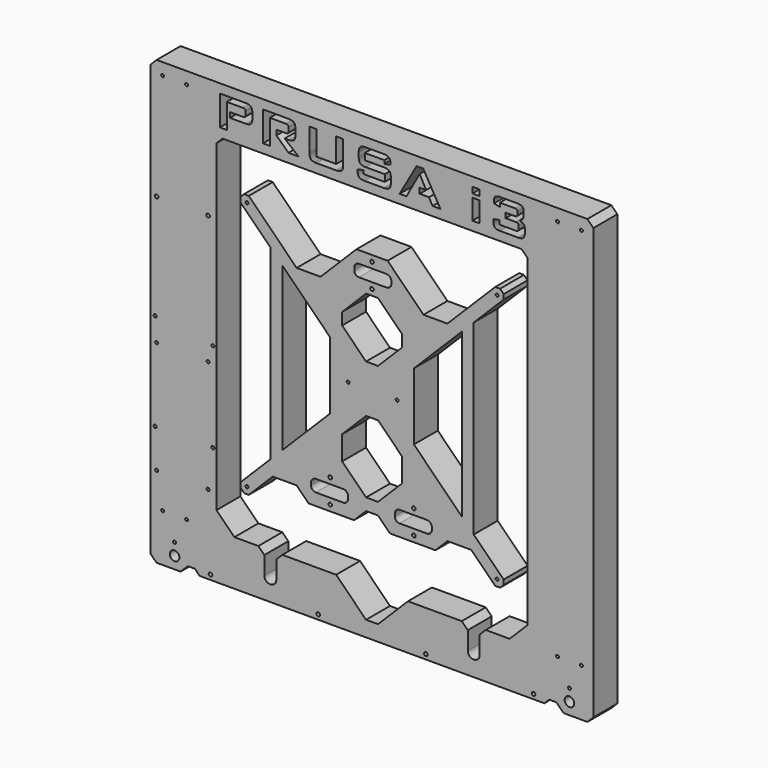
from build123d import *

# Parameters (mm, degrees)
F0_R     = 4
F0_R_2   = 1.2295
F0_R_3   = 1.5
F0_W     = 5.816832
F0_H     = 17
F0_H_2   = 5
F1_DEPTH = 25


# Not quite as in the source:
# - ends of sketch curves that miss each other by under 0.0002 mm in the source are joined


with BuildPart() as f1:
    # F0 (on Front) → F1 (new body)
    with BuildSketch(Plane.XZ):
        Polygon((338.0000003539, 10.00000019), (344.0000003539, 10.00000019), (350.0000003539, 4.00000019), (370.0000003539, 4.00000019), (375.0000003539, 9.00000019), (375.0000003539, 369.00000019), (370.0000003539, 374.00000019), (10.0000003539, 374.00000019), (5.0000003539, 369.00000019), (5.0000003539, 8.80825219), (10.0000003539, 4.00000019), (30.0000003539, 4.00000019), (36.0000003539, 10.00000019), (42.0000003539, 10.00000019), (46.0000003539, 6.00000019), (334.0000003539, 6.00000019), align=None)
        with Locations((25.0000003539, 14.00000019)):
            Circle(F0_R, mode=Mode.SUBTRACT)
        with Locations((25.0000003539, 24.00000019)):
            Circle(F0_R_2, mode=Mode.SUBTRACT)
        with Locations((15.0000003539, 44.00000019)):
            Circle(F0_R_2, mode=Mode.SUBTRACT)
        with Locations((35.0000003539, 44.00000019)):
            Circle(F0_R_2, mode=Mode.SUBTRACT)
        with Locations((55.0000003539, 10.00000019)):
            Circle(F0_R_3, mode=Mode.SUBTRACT)
        with Locations((10.0000003539, 72.00000019)):
            Circle(F0_R_2, mode=Mode.SUBTRACT)
        with Locations((53.0000003539, 72.00000019)):
            Circle(F0_R_2, mode=Mode.SUBTRACT)
        with Locations((145.0000003539, 10.00000019)):
            Circle(F0_R_3, mode=Mode.SUBTRACT)
        with Locations((8.7400003539, 104.00000019)):
            Circle(F0_R_2, mode=Mode.SUBTRACT)
        with Locations((57.0000003539, 104.00000019)):
            Circle(F0_R_2, mode=Mode.SUBTRACT)
        with Locations((10.0000003539, 166.00000019)):
            Circle(F0_R_2, mode=Mode.SUBTRACT)
        with Locations((8.7400003539, 185.28000019)):
            Circle(F0_R_2, mode=Mode.SUBTRACT)
        with Locations((53.0000003539, 166.00000019)):
            Circle(F0_R_2, mode=Mode.SUBTRACT)
        with Locations((57.0000003539, 178.93000019)):
            Circle(F0_R_2, mode=Mode.SUBTRACT)
        with BuildLine():
            Line((60.0000003539, 59.00000019), (60.0000003539, 329.00000019))
            Line((60.0000003539, 329.00000019), (65.0000003539, 334.00000019))
            Line((65.0000003539, 334.00000019), (315.0000003539, 334.00000019))
            Line((315.0000003539, 334.00000019), (320.0000003539, 329.00000019))
            Line((320.0000003539, 329.00000019), (320.0000003539, 59.00000019))
            Line((320.0000003539, 59.00000019), (305.0000003539, 44.00000019))
            Line((305.0000003539, 44.00000019), (285.0000003539, 44.00000019))
            Line((285.0000003539, 44.00000019), (280.0000003539, 39.00000019))
            Line((280.0000003539, 39.00000019), (280.0000003539, 24.00000019))
            ThreePointArc((280.0000003539, 24.00000019), (275.0000003539, 19.00000019), (270.0000003539, 24.00000019))
            Line((270.0000003539, 24.00000019), (270.0000003539, 39.00000019))
            Line((270.0000003539, 39.00000019), (265.0000003539, 44.00000019))
            Line((265.0000003539, 44.00000019), (220.0000003539, 44.00000019))
            Line((220.0000003539, 44.00000019), (195.0000003539, 19.00000019))
            Line((195.0000003539, 19.00000019), (185.0000003539, 19.00000019))
            Line((185.0000003539, 19.00000019), (160.0000003539, 44.00000019))
            Line((160.0000003539, 44.00000019), (115.0000003539, 44.00000019))
            Line((115.0000003539, 44.00000019), (110.0000003539, 39.00000019))
            Line((110.0000003539, 39.00000019), (110.0000003539, 24.00000019))
            ThreePointArc((110.0000003539, 24.00000019), (105.0000003539, 19.00000019), (100.0000003539, 24.00000019))
            Line((100.0000003539, 24.00000019), (100.0000003539, 39.00000019))
            Line((100.0000003539, 39.00000019), (95.0000003539, 44.00000019))
            Line((95.0000003539, 44.00000019), (75.0000003539, 44.00000019))
            Line((75.0000003539, 44.00000019), (65.0000003539, 54.00000019))
            Line((65.0000003539, 54.00000019), (60.0000003539, 59.00000019))
        make_face(mode=Mode.SUBTRACT)
        with Locations((235.0000003539, 10.00000019)):
            Circle(F0_R_3, mode=Mode.SUBTRACT)
        with Locations((325.0000003539, 10.00000019)):
            Circle(F0_R_3, mode=Mode.SUBTRACT)
        with Locations((355.0000003539, 14.00000019)):
            Circle(F0_R, mode=Mode.SUBTRACT)
        with Locations((355.0000003539, 24.00000019)):
            Circle(F0_R_2, mode=Mode.SUBTRACT)
        with Locations((345.0000003539, 44.00000019)):
            Circle(F0_R_2, mode=Mode.SUBTRACT)
        with Locations((365.0000003539, 44.00000019)):
            Circle(F0_R_2, mode=Mode.SUBTRACT)
        with Locations((10.0000003539, 273.50000019)):
            Circle(F0_R_3, mode=Mode.SUBTRACT)
        with Locations((53.0000003539, 273.50000019)):
            Circle(F0_R_3, mode=Mode.SUBTRACT)
        with Locations((15.0000003539, 364.00000019)):
            Circle(F0_R_2, mode=Mode.SUBTRACT)
        with Locations((35.0000003539, 364.00000019)):
            Circle(F0_R_2, mode=Mode.SUBTRACT)
        Polygon((81.6980203539, 362.16831719), (68.6039603539, 362.16831719), (68.6039603539, 341.50000019), (62.8861393539, 341.50000019), (62.8861393539, 366.50000019), (84.2722773539, 366.50000019), (84.7559833539, 366.49198919), (85.2169993539, 366.46803319), (85.6553223539, 366.42805519), (86.0709573539, 366.37209319), (86.4639043539, 366.30018619), (86.8341593539, 366.21225719), (87.1817263539, 366.10834519), (87.5065993539, 365.98844919), (87.8087853539, 365.85257019), (88.0882843539, 365.70070619), (88.3450893539, 365.53286019), (88.5792063539, 365.34899119), (88.7926963539, 365.14746119), (88.9876223539, 364.92651419), (89.1639853539, 364.68611119), (89.3217803539, 364.42629219), (89.4610173539, 364.14705719), (89.5816853539, 363.84840419), (89.6837853539, 363.53029619), (89.7673273539, 363.19281019), (89.8323013539, 362.83586919), (89.8787123539, 362.45951119), (89.9065593539, 362.06373619), (89.9158433539, 361.64850619), (89.9158423539, 356.07920819), (89.9065593539, 355.66793819), (89.8787123539, 355.27578719), (89.8323013539, 354.90271019), (89.7673273539, 354.54866819), (89.6837853539, 354.21373719), (89.5816853539, 353.89788119), (89.4610173539, 353.60113519), (89.3217803539, 353.32342519), (89.1639853539, 353.06482719), (88.9876223539, 352.82530219), (88.7926963539, 352.60485119), (88.5792063539, 352.40347319), (88.3450893539, 352.21964319), (88.0882843539, 352.05175819), (87.8087853539, 351.89989519), (87.5065993539, 351.76401519), (87.1817263539, 351.64411919), (86.8341593539, 351.54020719), (86.4639043539, 351.45231619), (86.0709573539, 351.38037119), (85.6553223539, 351.32440919), (85.2169993539, 351.28443119), (84.7559833539, 351.26047519), (84.2722753539, 351.25246419), (71.2539603539, 351.25247519), (71.2539603539, 355.55940619), (81.6980203539, 355.55940619), (81.9430543539, 355.56242419), (82.1748503539, 355.57142619), (82.3934083539, 355.58649419), (82.5987343539, 355.60755219), (82.7908233539, 355.63459819), (82.9696803539, 355.66770919), (83.1352953539, 355.70681019), (83.2876783539, 355.75193819), (83.4268243539, 355.80305519), (83.5527373539, 355.86019919), (83.6654143539, 355.92337019), (83.7648533539, 355.99256919), (83.8538073539, 356.06951119), (83.9350273539, 356.15587619), (84.0085083539, 356.25170119), (84.0742593539, 356.35698719), (84.1322713539, 356.47173319), (84.1825493539, 356.59590119), (84.2250923539, 356.72956819), (84.2599013539, 356.87265819), (84.2869763539, 357.02520819), (84.3063123539, 357.18721819), (84.3179133539, 357.35868819), (84.3217803539, 357.53961919), (84.3217823539, 360.21287119), (84.3179133539, 360.38984719), (84.3063123539, 360.55769319), (84.2869763539, 360.71642319), (84.2599013539, 360.86607419), (84.2250923539, 361.00656919), (84.1825493539, 361.13798519), (84.1322713539, 361.26028419), (84.0742593539, 361.37350519), (84.0085083539, 361.47757019), (83.9350273539, 361.57255619), (83.8538073539, 361.65838619), (83.7648533539, 361.73513819), (83.6654143539, 361.80433719), (83.5527373539, 361.86750819), (83.4268243539, 361.92465219), (83.2876783539, 361.97580719), (83.1352953539, 362.02093519), (82.9696803539, 362.06003619), (82.7908233539, 362.09310919), (82.5987343539, 362.12019319), (82.3934083539, 362.14125119), (82.1748503539, 362.15628119), (81.9430543539, 362.16532119), align=None, mode=Mode.SUBTRACT)
        Polygon((117.6881193539, 362.16831719), (104.5940593539, 362.16831719), (104.5940593539, 341.50000019), (98.8762383539, 341.50000019), (98.8762383539, 366.50000019), (120.2623763539, 366.50000019), (120.7460783539, 366.49198919), (121.2070943539, 366.46803319), (121.6454223539, 366.42805519), (122.0610523539, 366.37209319), (122.4540043539, 366.30018619), (122.8242593539, 366.21225719), (123.1718253539, 366.10834519), (123.4967043539, 365.98844919), (123.7988853539, 365.85257019), (124.0783793539, 365.70070619), (124.3351943539, 365.53286019), (124.5693113539, 365.34899119), (124.7828013539, 365.14746119), (124.9777223539, 364.92651419), (125.1540853539, 364.68611119), (125.3118803539, 364.42629219), (125.4511173539, 364.14705719), (125.5717853539, 363.84840419), (125.6738853539, 363.53029619), (125.7574273539, 363.19281019), (125.8224013539, 362.83586919), (125.8688163539, 362.45951119), (125.8966543539, 362.06373619), (125.9059433539, 361.64850619), (125.9059413539, 355.80693119), (125.8966543539, 355.39560719), (125.8688163539, 355.00315119), (125.8224013539, 354.62965419), (125.7574273539, 354.27504019), (125.6738853539, 353.93930819), (125.5717853539, 353.62253619), (125.4511173539, 353.32464619), (125.3118803539, 353.04563919), (125.1540853539, 352.78559119), (124.9777223539, 352.54442619), (124.7828013539, 352.32214419), (124.5693113539, 352.11882019), (124.3351943539, 351.93300619), (124.0783793539, 351.76332919), (123.7988853539, 351.60982519), (123.4967043539, 351.47249619), (123.1718253539, 351.35130319), (122.8242593539, 351.24628419), (122.4540043539, 351.15740219), (122.0610523539, 351.08469419), (121.6454223539, 351.02816019), (121.2070943539, 350.98776219), (120.7460783539, 350.96353919), (120.2623753539, 350.95545219), (116.9950503539, 350.95544619), (128.5297033539, 341.50000019), (120.1881193539, 341.50000019), (110.1138613539, 350.95544619), (110.1138613539, 355.23762419), (117.6881193539, 355.23762419), (117.9331493539, 355.24061619), (118.1649493539, 355.24965719), (118.3835123539, 355.26468719), (118.5888393539, 355.28574419), (118.7809283539, 355.31282819), (118.9597803539, 355.34590119), (119.1253953539, 355.38504019), (119.2777823539, 355.43013019), (119.4169243539, 355.48128519), (119.5428373539, 355.53842919), (119.6555143539, 355.60160119), (119.7549533539, 355.67079919), (119.8439033539, 355.74770419), (119.9251273539, 355.83410619), (119.9986083539, 355.92993219), (120.0643543539, 356.03521719), (120.1223663539, 356.14992519), (120.1726533539, 356.27413219), (120.2151873539, 356.40779919), (120.2499963539, 356.55088819), (120.2770713539, 356.70343819), (120.2964123539, 356.86544819), (120.3080183539, 357.03691919), (120.3118803539, 357.21781219), (120.3118813539, 360.21287119), (120.3080183539, 360.38984719), (120.2964123539, 360.55769319), (120.2770713539, 360.71642319), (120.2499963539, 360.86607419), (120.2151873539, 361.00656919), (120.1726533539, 361.13798519), (120.1223663539, 361.26028419), (120.0643543539, 361.37350519), (119.9986083539, 361.47757019), (119.9251273539, 361.57255619), (119.8439033539, 361.65838619), (119.7549533539, 361.73513819), (119.6555143539, 361.80433719), (119.5428373539, 361.86750819), (119.4169243539, 361.92465219), (119.2777823539, 361.97580719), (119.1253953539, 362.02093519), (118.9597803539, 362.06003619), (118.7809283539, 362.09310919), (118.5888393539, 362.12019319), (118.3835123539, 362.14125119), (118.1649493539, 362.15628119), (117.9331493539, 362.16532119), align=None, mode=Mode.SUBTRACT)
        Polygon((137.6881193539, 347.41584219), (137.6881193539, 366.50000019), (143.5049503539, 366.50000019), (143.5049503539, 346.20297019), (160.0643563539, 346.20297019), (160.0643563539, 366.50000019), (165.8564363539, 366.50000019), (165.8564363539, 347.41584219), (165.8475883539, 346.85770419), (165.8210283539, 346.33017019), (165.7767683539, 345.83322919), (165.7147983539, 345.36688219), (165.6351283539, 344.93112919), (165.5377483539, 344.52600919), (165.4226683539, 344.15144319), (165.2898793539, 343.80747219), (165.1393893539, 343.49413319), (164.9711893539, 343.21134919), (164.7852903539, 342.95919819), (164.5816803539, 342.73764019), (164.3528083539, 342.53996319), (164.0911013539, 342.35945119), (163.7965683539, 342.19618219), (163.4692003539, 342.05004119), (163.1089973539, 341.92114319), (162.7159693539, 341.80941019), (162.2901063539, 341.71488219), (161.8314083539, 341.63752019), (161.3398843539, 341.57736219), (160.8155253539, 341.53437019), (160.2583413539, 341.50858319), (159.6683123539, 341.50000019), (143.8762383539, 341.50000019), (143.2900813539, 341.50858319), (142.7362443539, 341.53437019), (142.2147273539, 341.57736219), (141.7255213539, 341.63752019), (141.2686353539, 341.71488219), (140.8440593539, 341.80941019), (140.4518033539, 341.92114319), (140.0918583539, 342.05004119), (139.7642333539, 342.19618219), (139.4689183539, 342.35945119), (139.2059233539, 342.53996319), (138.9752483539, 342.73764019), (138.7696653539, 342.95919819), (138.5819633539, 343.21134919), (138.4121323539, 343.49413319), (138.2601743539, 343.80747219), (138.1260973539, 344.15144319), (138.0099013539, 344.52600919), (137.9115773539, 344.93112919), (137.8311353539, 345.36688219), (137.7685643539, 345.83322919), (137.7238753539, 346.33017019), (137.6970583539, 346.85770419), align=None, mode=Mode.SUBTRACT)
        Polygon((205.4108913539, 360.48514919), (200.2871293539, 359.27227719), (200.2871293539, 362.11881219), (183.9257433539, 362.11881219), (183.9257433539, 356.74752519), (199.4950503539, 356.74752519), (200.0930603539, 356.73883819), (200.6577303539, 356.71278419), (201.1890413539, 356.66941119), (201.6870123539, 356.60864319), (202.1516423539, 356.53051819), (202.5829123539, 356.43503619), (202.9808433539, 356.32215919), (203.3454323539, 356.19196319), (203.6766623539, 356.04441119), (203.9745523539, 355.87946319), (204.2391013539, 355.69715919), (204.4702913539, 355.49753619), (204.6758843539, 355.27414719), (204.8635863539, 355.02069919), (205.0334173539, 354.73715219), (205.1853753539, 354.42354619), (205.3194433539, 354.07984219), (205.4356383539, 353.70607819), (205.5339623539, 353.30221619), (205.6144143539, 352.86825619), (205.6769753539, 352.40423619), (205.7216643539, 351.91011819), (205.7484823539, 351.38594119), (205.7574273539, 350.83166519), (205.7574263539, 347.41584219), (205.7484823539, 346.86155719), (205.7216643539, 346.33737919), (205.6769753539, 345.84330019), (205.6144143539, 345.37928019), (205.5339623539, 344.94532019), (205.4356383539, 344.54145819), (205.3194433539, 344.16769419), (205.1853753539, 343.82399019), (205.0334173539, 343.51038419), (204.8635863539, 343.22683719), (204.6758843539, 342.97338919), (204.4702913539, 342.75000019), (204.2391013539, 342.55033919), (203.9745523539, 342.36807319), (203.6766623539, 342.20312519), (203.3454323539, 342.05557319), (202.9808433539, 341.92533919), (202.5829123539, 341.81250019), (202.1516423539, 341.71701819), (201.6870123539, 341.63889319), (201.1890413539, 341.57812519), (200.6577303539, 341.53471419), (200.0930603539, 341.50869819), (199.4950493539, 341.50000019), (184.0742573539, 341.50000019), (183.4801963539, 341.50869819), (182.9191403539, 341.53471419), (182.3910903539, 341.57812519), (181.8960383539, 341.63889319), (181.4339923539, 341.71701819), (181.0049533539, 341.81250019), (180.6089123539, 341.92533919), (180.2458763539, 342.05557319), (179.9158383539, 342.20312519), (179.6188163539, 342.36807319), (179.3547823539, 342.55033919), (179.1237643539, 342.75000019), (178.9181803539, 342.97338919), (178.7304693539, 343.22683719), (178.5606483539, 343.51038419), (178.4086893539, 343.82399019), (178.2746123539, 344.16769419), (178.1584173539, 344.54145819), (178.0600933539, 344.94532019), (177.9796503539, 345.37928019), (177.9170803539, 345.84330019), (177.8723913539, 346.33737919), (177.8455733539, 346.86155719), (177.8366373539, 347.41583319), (177.8366343539, 348.08415819), (182.9603963539, 349.14851519), (182.9603963539, 346.20297019), (200.6336633539, 346.20297019), (200.6336633539, 351.89604019), (185.0396043539, 351.89604019), (184.4495873539, 351.90470119), (183.8923933539, 351.93075619), (183.3680343539, 351.97416719), (182.8765113539, 352.03493519), (182.4178223539, 352.11306019), (181.9919593539, 352.20854219), (181.5989213539, 352.32138119), (181.2387283539, 352.45157619), (180.9113603539, 352.59916719), (180.6168173539, 352.76407619), (180.3551103539, 352.94638119), (180.1262383539, 353.14604219), (179.9226283539, 353.36943119), (179.7367293539, 353.62287919), (179.5685293539, 353.90638719), (179.4180393539, 354.22003219), (179.2852593539, 354.56373619), (179.1701703539, 354.93750019), (179.0728003539, 355.34136219), (178.9931203539, 355.77528419), (178.9311603539, 356.23934219), (178.8868903539, 356.73342119), (178.8603403539, 357.25759919), (178.8514803539, 357.81187419), (178.8514853539, 360.58415819), (178.8603403539, 361.13844319), (178.8868903539, 361.66262119), (178.9311603539, 362.15670019), (178.9931203539, 362.62072019), (179.0728003539, 363.05468019), (179.1701703539, 363.45854219), (179.2852593539, 363.83230619), (179.4180393539, 364.17601019), (179.5685293539, 364.48961619), (179.7367293539, 364.77316319), (179.9226283539, 365.02661119), (180.1262383539, 365.25000019), (180.3551103539, 365.44966119), (180.6168173539, 365.63192719), (180.9113603539, 365.79687519), (181.2387283539, 365.94442719), (181.5989213539, 366.07466119), (181.9919593539, 366.18750019), (182.4178223539, 366.28298219), (182.8765113539, 366.36110719), (183.3680343539, 366.42187519), (183.8923933539, 366.46528619), (184.4495873539, 366.49130219), (185.0395973539, 366.50000019), (199.2227723539, 366.50000019), (199.7934533539, 366.49157019), (200.3338813539, 366.46631619), (200.8440593539, 366.42420219), (201.3239863539, 366.36522719), (201.7736433539, 366.28942919), (202.1930693539, 366.19677019), (202.5822263539, 366.08728819), (202.9411513539, 365.96094519), (203.2698063539, 365.81774119), (203.5682113539, 365.65771519), (203.8363653539, 365.48086519), (204.0742493539, 365.28711719), (204.2877393539, 365.07208319), (204.4826703539, 364.83126119), (204.6590423539, 364.56465119), (204.8168373539, 364.27229319), (204.9560743539, 363.95410919), (205.0767333539, 363.61013819), (205.1788333539, 363.24041719), (205.2623753539, 362.84487219), (205.3273583539, 362.42357619), (205.3737643539, 361.97649419), (205.4016113539, 361.50362419), (205.4109003539, 361.00496719), align=None, mode=Mode.SUBTRACT)
        Polygon((229.7920793539, 351.47524819), (235.1881193539, 351.47524819), (229.7920793539, 361.64851519), (224.2475253539, 351.47524819), (221.7475253539, 346.97029719), (218.8514853539, 341.50000019), (213.0594063539, 341.50000019), (227.1930693539, 366.50000019), (232.7871293539, 366.50000019), (247.1188123539, 341.50000019), (240.5841583539, 341.50000019), (237.5891093539, 346.97029719), (229.7920793539, 346.97029719), align=None, mode=Mode.SUBTRACT)
        with Locations((276.8094063539, 350.00000019)):
            Rectangle(F0_W, F0_H, mode=Mode.SUBTRACT)
        with Locations((276.8094063539, 364.00000019)):
            Rectangle(F0_W, F0_H_2, mode=Mode.SUBTRACT)
        with BuildLine():
            Line((312.2241023539, 341.50801119), (311.6732603539, 341.50000019))
            Line((311.6732603539, 341.50000019), (297.1435643539, 341.50000019))
            Line((297.1435643539, 341.50000019), (296.5977293539, 341.50721019))
            Line((296.5977293539, 341.50721019), (296.0823063539, 341.52887719))
            Line((296.0823063539, 341.52887719), (295.5973053539, 341.56496419))
            Line((295.5973053539, 341.56496419), (295.1427463539, 341.61550919))
            Line((295.1427463539, 341.61550919), (294.7185903539, 341.68047319))
            Line((294.7185903539, 341.68047319), (294.3248753539, 341.75989519))
            Line((294.3248753539, 341.75989519), (293.9615823539, 341.85373719))
            Line((293.9615823539, 341.85373719), (293.6287123539, 341.96203619))
            Line((293.6287123539, 341.96203619), (293.3262633539, 342.08479319))
            Line((293.3262633539, 342.08479319), (293.0542563539, 342.22193119))
            Line((293.0542563539, 342.22193119), (292.8126533539, 342.37356619))
            Line((292.8126533539, 342.37356619), (292.6014903539, 342.53961919))
            Line((292.6014903539, 342.53961919), (292.4136923539, 342.72509019))
            Line((292.4136923539, 342.72509019), (292.2422223539, 342.93497519))
            Line((292.2422223539, 342.93497519), (292.0870973539, 343.16923519))
            Line((292.0870973539, 343.16923519), (291.9482993539, 343.42794819))
            Line((291.9482993539, 343.42794819), (291.8258293539, 343.71103719))
            Line((291.8258293539, 343.71103719), (291.7196853539, 344.01857819))
            Line((291.7196853539, 344.01857819), (291.6298683539, 344.35049419))
            Line((291.6298683539, 344.35049419), (291.5563773539, 344.70682519))
            Line((291.5563773539, 344.70682519), (291.4992333539, 345.08757019))
            Line((291.4992333539, 345.08757019), (291.4583973539, 345.49272919))
            Line((291.4583973539, 345.49272919), (291.4339073539, 345.92226419))
            Line((291.4339073539, 345.92226419), (291.4257433539, 346.37625119))
            Line((291.4257433539, 346.37625119), (291.4257433539, 348.43069319))
            Line((291.4257433539, 348.43069319), (296.5495053539, 349.49505019))
            Line((296.5495053539, 349.49505019), (296.5495053539, 345.98019819))
            Line((296.5495053539, 345.98019819), (310.0396043539, 345.98019819))
            Line((310.0396043539, 345.98019819), (310.2722553539, 345.98329919))
            Line((310.2722553539, 345.98329919), (310.4916763539, 345.99256919))
            Line((310.4916763539, 345.99256919), (310.6978613539, 346.00805719))
            Line((310.6978613539, 346.00805719), (310.8908083539, 346.02968619))
            Line((310.8908083539, 346.02968619), (311.0705183539, 346.05753319))
            Line((311.0705183539, 346.05753319), (311.2370113539, 346.09159919))
            Line((311.2370113539, 346.09159919), (311.3902473539, 346.13180519))
            Line((311.3902473539, 346.13180519), (311.5302473539, 346.17823019))
            Line((311.5302473539, 346.17823019), (311.6570283539, 346.23083519))
            Line((311.6570283539, 346.23083519), (311.7705543539, 346.28961919))
            Line((311.7705543539, 346.28961919), (311.8708613539, 346.35458419))
            Line((311.8708613539, 346.35458419), (311.9579123539, 346.42572819))
            Line((311.9579123539, 346.42572819), (312.0350073539, 346.50637119))
            Line((312.0350073539, 346.50637119), (312.1054083539, 346.59971619))
            Line((312.1054083539, 346.59971619), (312.1690943539, 346.70576519))
            Line((312.1690943539, 346.70576519), (312.2260673539, 346.82451619))
            Line((312.2260673539, 346.82451619), (312.2763443539, 346.95604719))
            Line((312.2763443539, 346.95604719), (312.3199273539, 347.10024319))
            Line((312.3199273539, 347.10024319), (312.3567963539, 347.25717919))
            Line((312.3567963539, 347.25717919), (312.3869713539, 347.42685719))
            Line((312.3869713539, 347.42685719), (312.4104313539, 347.60923819))
            Line((312.4104313539, 347.60923819), (312.4271773539, 347.80432119))
            Line((312.4271773539, 347.80432119), (312.4372483539, 348.01214619))
            Line((312.4372483539, 348.01214619), (312.4405863539, 348.23267419))
            Line((312.4405863539, 348.23267419), (312.4405943539, 350.06435619))
            Line((312.4405943539, 350.06435619), (312.4371533539, 350.28894819))
            Line((312.4371533539, 350.28894819), (312.4268343539, 350.50062619))
            Line((312.4268343539, 350.50062619), (312.4096493539, 350.69940919))
            Line((312.4096493539, 350.69940919), (312.3855973539, 350.88530019))
            Line((312.3855973539, 350.88530019), (312.3546413539, 351.05833419))
            Line((312.3546413539, 351.05833419), (312.3168373539, 351.21843719))
            Line((312.3168373539, 351.21843719), (312.2721483539, 351.36568519))
            Line((312.2721483539, 351.36568519), (312.2205733539, 351.50000019))
            Line((312.2205733539, 351.50000019), (312.1621323539, 351.62146019))
            Line((312.1621323539, 351.62146019), (312.0968063539, 351.72998819))
            Line((312.0968063539, 351.72998819), (312.0246123539, 351.82566119))
            Line((312.0246123539, 351.82566119), (311.9455533539, 351.90840119))
            Line((311.9455533539, 351.90840119), (311.8566703539, 351.98156719))
            Line((311.8566703539, 351.98156719), (311.7550853539, 352.04832519))
            Line((311.7550853539, 352.04832519), (311.6407783539, 352.10874919))
            Line((311.6407783539, 352.10874919), (311.5137483539, 352.16280419))
            Line((311.5137483539, 352.16280419), (311.3739973539, 352.21052619))
            Line((311.3739973539, 352.21052619), (311.2215423539, 352.25183919))
            Line((311.2215423539, 352.25183919), (311.0563473539, 352.28681919))
            Line((311.0563473539, 352.28681919), (310.8784293539, 352.31546819))
            Line((310.8784293539, 352.31546819), (310.6878093539, 352.33770819))
            Line((310.6878093539, 352.33770819), (310.4844673539, 352.35361519))
            Line((310.4844673539, 352.35361519), (310.2683833539, 352.36315219))
            Line((310.2683833539, 352.36315219), (310.0395973539, 352.36631819))
            Line((310.0395973539, 352.36631819), (301.5990103539, 352.36633719))
            Line((301.5990103539, 352.36633719), (301.5990103539, 356.42574319))
            Line((301.5990103539, 356.42574319), (309.1237623539, 356.42574319))
            Line((309.1237623539, 356.42574319), (309.3523793539, 356.42881819))
            Line((309.3523793539, 356.42881819), (309.5679283539, 356.43812619))
            Line((309.5679283539, 356.43812619), (309.7704123539, 356.45357519))
            Line((309.7704123539, 356.45357519), (309.9598503539, 356.47524319))
            Line((309.9598503539, 356.47524319), (310.1362043539, 356.50309019))
            Line((310.1362043539, 356.50309019), (310.2995113539, 356.53711719))
            Line((310.2995113539, 356.53711719), (310.4497343539, 356.57736219))
            Line((310.4497343539, 356.57736219), (310.5869103539, 356.62374919))
            Line((310.5869103539, 356.62374919), (310.7110213539, 356.67635319))
            Line((310.7110213539, 356.67635319), (310.8220483539, 356.73513819))
            Line((310.8220483539, 356.73513819), (310.9200293539, 356.80014019))
            Line((310.9200293539, 356.80014019), (311.0049443539, 356.87128419))
            Line((311.0049443539, 356.87128419), (311.0800743539, 356.95208019))
            Line((311.0800743539, 356.95208019), (311.1486433539, 357.04592119))
            Line((311.1486433539, 357.04592119), (311.2107093539, 357.15284719))
            Line((311.2107093539, 357.15284719), (311.2662323539, 357.27282019))
            Line((311.2662323539, 357.27282019), (311.3152123539, 357.40587619))
            Line((311.3152123539, 357.40587619), (311.3576703539, 357.55197919))
            Line((311.3576703539, 357.55197919), (311.3936043539, 357.71116619))
            Line((311.3936043539, 357.71116619), (311.4229973539, 357.88340019))
            Line((311.4229973539, 357.88340019), (311.4458473539, 358.06868019))
            Line((311.4458473539, 358.06868019), (311.4621933539, 358.26704419))
            Line((311.4621933539, 358.26704419), (311.4719773539, 358.47849319))
            Line((311.4719773539, 358.47849319), (311.4752393539, 358.70298819))
            Line((311.4752393539, 358.70298819), (311.4752483539, 359.94059419))
            Line((311.4752483539, 359.94059419), (311.4719773539, 360.16905219))
            Line((311.4719773539, 360.16905219), (311.4621933539, 360.38408719))
            Line((311.4621933539, 360.38408719), (311.4458473539, 360.58569319))
            Line((311.4458473539, 360.58569319), (311.4229973539, 360.77391119))
            Line((311.4229973539, 360.77391119), (311.3936043539, 360.94873819))
            Line((311.3936043539, 360.94873819), (311.3576703539, 361.11013819))
            Line((311.3576703539, 361.11013819), (311.3152123539, 361.25814819))
            Line((311.3152123539, 361.25814819), (311.2662323539, 361.39273119))
            Line((311.2662323539, 361.39273119), (311.2107093539, 361.51392419))
            Line((311.2107093539, 361.51392419), (311.1486433539, 361.62168919))
            Line((311.1486433539, 361.62168919), (311.0800743539, 361.71606419))
            Line((311.0800743539, 361.71606419), (311.0049443539, 361.79701219))
            Line((311.0049443539, 361.79701219), (310.9200293539, 361.86819519))
            Line((310.9200293539, 361.86819519), (310.8220483539, 361.93315919))
            Line((310.8220483539, 361.93315919), (310.7110213539, 361.99194319))
            Line((310.7110213539, 361.99194319), (310.5869103539, 362.04454819))
            Line((310.5869103539, 362.04454819), (310.4497343539, 362.09097319))
            Line((310.4497343539, 362.09097319), (310.2995113539, 362.13118019))
            Line((310.2995113539, 362.13118019), (310.1362043539, 362.16520719))
            Line((310.1362043539, 362.16520719), (309.9598503539, 362.19305419))
            Line((309.9598503539, 362.19305419), (309.7704123539, 362.21472219))
            Line((309.7704123539, 362.21472219), (309.5679283539, 362.23020919))
            Line((309.5679283539, 362.23020919), (309.3523793539, 362.23947919))
            Line((309.3523793539, 362.23947919), (309.1237643539, 362.24256919))
            Line((309.1237643539, 362.24256919), (296.7722773539, 362.24257419))
            Line((296.7722773539, 362.24257419), (296.7722773539, 359.12376219))
            Line((296.7722773539, 359.12376219), (291.8217823539, 360.03960419))
            Line((291.8217823539, 360.03960419), (291.8217823539, 361.59901019))
            Line((291.8217823539, 361.59901019), (291.8298533539, 362.05694619))
            Line((291.8298533539, 362.05694619), (291.8540953539, 362.49010519))
            Line((291.8540953539, 362.49010519), (291.8944933539, 362.89850619))
            Line((291.8944933539, 362.89850619), (291.9510463539, 363.28218819))
            Line((291.9510463539, 363.28218819), (292.0237543539, 363.64107519))
            Line((292.0237543539, 363.64107519), (292.1126173539, 363.97524319))
            Line((292.1126173539, 363.97524319), (292.2176553539, 364.28465319))
            Line((292.2176553539, 364.28465319), (292.3388293539, 364.56930519))
            Line((292.3388293539, 364.56930519), (292.4761773539, 364.82920119))
            Line((292.4761773539, 364.82920119), (292.6296813539, 365.06433919))
            Line((292.6296813539, 365.06433919), (292.7993393539, 365.27475719))
            Line((292.7993393539, 365.27475719), (292.9851533539, 365.46038119))
            Line((292.9851533539, 365.46038119), (293.1945043539, 365.62643419))
            Line((293.1945043539, 365.62643419), (293.4348113539, 365.77806919))
            Line((293.4348113539, 365.77806919), (293.7060743539, 365.91520719))
            Line((293.7060743539, 365.91520719), (294.0082553539, 366.03796419))
            Line((294.0082553539, 366.03796419), (294.3413733539, 366.14626319))
            Line((294.3413733539, 366.14626319), (294.7054483539, 366.24010519))
            Line((294.7054483539, 366.24010519), (295.1004603539, 366.31952719))
            Line((295.1004603539, 366.31952719), (295.5264093539, 366.38449119))
            Line((295.5264093539, 366.38449119), (295.9832953539, 366.43503619))
            Line((295.9832953539, 366.43503619), (296.4711193539, 366.47112319))
            Line((296.4711193539, 366.47112319), (296.9898993539, 366.49279019))
            Line((296.9898993539, 366.49279019), (297.5395973539, 366.50000019))
            Line((297.5395973539, 366.50000019), (311.0544553539, 366.50000019))
            Line((311.0544553539, 366.50000019), (311.6002083539, 366.49279019))
            Line((311.6002083539, 366.49279019), (312.1153833539, 366.47112319))
            Line((312.1153833539, 366.47112319), (312.5999453539, 366.43503619))
            Line((312.5999453539, 366.43503619), (313.0539133539, 366.38449119))
            Line((313.0539133539, 366.38449119), (313.4772683539, 366.31952719))
            Line((313.4772683539, 366.31952719), (313.8700493539, 366.24010519))
            Line((313.8700493539, 366.24010519), (314.2322353539, 366.14626319))
            Line((314.2322353539, 366.14626319), (314.5638083539, 366.03796419))
            Line((314.5638083539, 366.03796419), (314.8647883539, 365.91520719))
            Line((314.8647883539, 365.91520719), (315.1351743539, 365.77806919))
            Line((315.1351743539, 365.77806919), (315.3749663539, 365.62643419))
            Line((315.3749663539, 365.62643419), (315.5841643539, 365.46038119))
            Line((315.5841643539, 365.46038119), (315.7699783539, 365.27475719))
            Line((315.7699783539, 365.27475719), (315.9396363539, 365.06433919))
            Line((315.9396363539, 365.06433919), (316.0931403539, 364.82920119))
            Line((316.0931403539, 364.82920119), (316.2304693539, 364.56930519))
            Line((316.2304693539, 364.56930519), (316.3516623539, 364.28465319))
            Line((316.3516623539, 364.28465319), (316.4566803539, 363.97524319))
            Line((316.4566803539, 363.97524319), (316.5455443539, 363.64107519))
            Line((316.5455443539, 363.64107519), (316.6182713539, 363.28218819))
            Line((316.6182713539, 363.28218819), (316.6748243539, 362.89850619))
            Line((316.6748243539, 362.89850619), (316.7152023539, 362.49010519))
            Line((316.7152023539, 362.49010519), (316.7394453539, 362.05694619))
            Line((316.7394453539, 362.05694619), (316.7475323539, 361.59899119))
            Line((316.7475323539, 361.59899119), (316.7475253539, 359.34653519))
            Line((316.7475253539, 359.34653519), (316.7401313539, 358.98729719))
            Line((316.7401313539, 358.98729719), (316.7179683539, 358.64382219))
            Line((316.7179683539, 358.64382219), (316.6810043539, 358.31621619))
            Line((316.6810043539, 358.31621619), (316.6292573539, 358.00440219))
            Line((316.6292573539, 358.00440219), (316.5627483539, 357.70842019))
            Line((316.5627483539, 357.70842019), (316.4814383539, 357.42823019))
            Line((316.4814383539, 357.42823019), (316.3853453539, 357.16383419))
            Line((316.3853453539, 357.16383419), (316.2744713539, 356.91530619))
            Line((316.2744713539, 356.91530619), (316.1488153539, 356.68253319))
            Line((316.1488153539, 356.68253319), (316.0083963539, 356.46563019))
            Line((316.0083963539, 356.46563019), (315.8531763539, 356.26451919))
            Line((315.8531763539, 356.26451919), (315.6831743539, 356.07920119))
            Line((315.6831743539, 356.07920119), (315.4944233539, 355.90628119))
            Line((315.4944233539, 355.90628119), (315.2830123539, 355.74228719))
            Line((315.2830123539, 355.74228719), (315.0488853539, 355.58725719))
            Line((315.0488853539, 355.58725719), (314.7920803539, 355.44115419))
            Line((314.7920803539, 355.44115419), (314.5125773539, 355.30397819))
            Line((314.5125773539, 355.30397819), (314.2103963539, 355.17572819))
            Line((314.2103963539, 355.17572819), (313.7401013539, 355.00305019))
            ThreePointArc((313.7401013539, 355.00305019), (313.4857633539, 354.64797119), (313.7401014201, 354.2928923846))
            Line((313.7401014201, 354.2928923846), (314.1395003539, 354.18539419))
            Line((314.1395003539, 354.18539419), (314.5167163539, 354.06496419))
            Line((314.5167163539, 354.06496419), (314.8717503539, 353.93167919))
            Line((314.8717503539, 353.93167919), (315.2046203539, 353.78546119))
            Line((315.2046203539, 353.78546119), (315.5153083539, 353.62638919))
            Line((315.5153083539, 353.62638919), (315.8038333539, 353.45442219))
            Line((315.8038333539, 353.45442219), (316.0701753539, 353.26956219))
            Line((316.0701753539, 353.26956219), (316.3143543539, 353.07177019))
            Line((316.3143543539, 353.07177019), (316.5377243539, 352.85974919))
            Line((316.5377243539, 352.85974919), (316.7416763539, 352.63208819))
            Line((316.7416763539, 352.63208819), (316.9262123539, 352.38878619))
            Line((316.9262123539, 352.38878619), (317.0913123539, 352.12980719))
            Line((317.0913123539, 352.12980719), (317.2369963539, 351.85522519))
            Line((317.2369963539, 351.85522519), (317.3632433539, 351.56496419))
            Line((317.3632433539, 351.56496419), (317.4700743539, 351.25910219))
            Line((317.4700743539, 351.25910219), (317.5574873539, 350.93756119))
            Line((317.5574873539, 350.93756119), (317.6254653539, 350.60041819))
            Line((317.6254653539, 350.60041819), (317.6740263539, 350.24759719))
            Line((317.6740263539, 350.24759719), (317.7031523539, 349.87913519))
            Line((317.7031523539, 349.87913519), (317.7128793539, 349.49503319))
            Line((317.7128793539, 349.49503319), (317.7128713539, 346.87128719))
            Line((317.7128713539, 346.87128719), (317.7036673539, 346.37304719))
            Line((317.7036673539, 346.37304719), (317.6760863539, 345.90147419))
            Line((317.6760863539, 345.90147419), (317.6301003539, 345.45652819))
            Line((317.6301003539, 345.45652819), (317.5657273539, 345.03824619))
            Line((317.5657273539, 345.03824619), (317.4829673539, 344.64659119))
            Line((317.4829673539, 344.64659119), (317.3818023539, 344.28156319))
            Line((317.3818023539, 344.28156319), (317.2622493539, 343.94319919))
            Line((317.2622493539, 343.94319919), (317.1243103539, 343.63146219))
            Line((317.1243103539, 343.63146219), (316.9679833539, 343.34639019))
            Line((316.9679833539, 343.34639019), (316.7932513539, 343.08794419))
            Line((316.7932513539, 343.08794419), (316.6001323539, 342.85612519))
            Line((316.6001323539, 342.85612519), (316.3886073539, 342.65100919))
            Line((316.3886073539, 342.65100919), (316.1535453539, 342.46714019))
            Line((316.1535453539, 342.46714019), (315.8897783539, 342.29929419))
            Line((315.8897783539, 342.29929419), (315.5973053539, 342.14743019))
            Line((315.5973053539, 342.14743019), (315.2761273539, 342.01155119))
            Line((315.2761273539, 342.01155119), (314.9262433539, 341.89165519))
            Line((314.9262433539, 341.89165519), (314.5476533539, 341.78774319))
            Line((314.5476533539, 341.78774319), (314.1403583539, 341.69981419))
            Line((314.1403583539, 341.69981419), (313.7043383539, 341.62790719))
            Line((313.7043383539, 341.62790719), (313.2396323539, 341.57194519))
            Line((313.2396323539, 341.57194519), (312.7462203539, 341.53196719))
            Line((312.7462203539, 341.53196719), (312.2241023539, 341.50801119))
        make_face(mode=Mode.SUBTRACT)
        with Locations((345.0000003539, 364.00000019)):
            Circle(F0_R_2, mode=Mode.SUBTRACT)
        with Locations((365.0000003539, 364.00000019)):
            Circle(F0_R_2, mode=Mode.SUBTRACT)
    extrude(amount=F1_DEPTH)


with BuildPart() as f1b:
    # F0 (on Front) → F1, piece 2 (new body)
    with BuildSketch(Plane.XZ):
        Polygon((80.0000003539, 86.00000019), (80.0000003539, 82.00000019), (83.0000003539, 79.00000019), (87.0000003539, 79.00000019), (107.0000003539, 99.00000019), (127.0000003539, 99.00000019), (137.0000003539, 89.00000019), (175.0000003539, 89.00000019), (185.0000003539, 99.00000019), (195.0000003539, 99.00000019), (205.0000003539, 89.00000019), (243.0000003539, 89.00000019), (253.0000003539, 99.00000019), (273.0000003539, 99.00000019), (293.0000003539, 79.00000019), (297.0000003539, 79.00000019), (300.0000003539, 82.00000019), (300.0000003539, 86.00000019), (275.0000003539, 111.00000019), (275.0000003539, 267.00000019), (300.0000003539, 292.00000019), (300.0000003539, 296.00000019), (297.0000003539, 299.00000019), (293.0000003539, 299.00000019), (253.0000003539, 259.00000019), (233.0000003539, 259.00000019), (203.0000003539, 289.00000019), (177.0000003539, 289.00000019), (147.0000003539, 259.00000019), (127.0000003539, 259.00000019), (87.0000003539, 299.00000019), (83.0000003539, 299.00000019), (80.0000003539, 296.00000019), (80.0000003539, 292.00000019), (105.0000003539, 267.00000019), (105.0000003539, 111.00000019), align=None)
        with Locations((85.5000003539, 84.50000019)):
            Circle(F0_R_2, mode=Mode.SUBTRACT)
        with Locations((155.0000003539, 94.00000019)):
            Circle(F0_R_3, mode=Mode.SUBTRACT)
        with BuildLine():
            ThreePointArc((169.9929633539, 103.00000019), (168.8213904786, 100.1715730652), (165.9929633539, 99.00000019))
            Line((165.9929633539, 99.00000019), (142.9929633539, 99.00000019))
            ThreePointArc((142.9929633539, 99.00000019), (140.1645362292, 100.1715730652), (138.9929633539, 103.00000019))
            Line((138.9929633539, 103.00000019), (138.9929633539, 105.00000019))
            ThreePointArc((138.9929633539, 105.00000019), (140.1645362292, 107.8284273147), (142.9929633539, 109.00000019))
            Line((142.9929633539, 109.00000019), (165.9929633539, 109.00000019))
            ThreePointArc((165.9929633539, 109.00000019), (168.8213904786, 107.8284273147), (169.9929633539, 105.00000019))
            Line((169.9929633539, 105.00000019), (169.9929633539, 103.00000019))
        make_face(mode=Mode.SUBTRACT)
        with Locations((155.0000003539, 114.00000019)):
            Circle(F0_R_3, mode=Mode.SUBTRACT)
        Polygon((215.0000003539, 129.00000019), (195.0000003539, 109.00000019), (185.0000003539, 109.00000019), (165.0000003539, 129.00000019), (165.0000003539, 149.00000019), (185.0000003539, 169.00000019), (195.0000003539, 169.00000019), (215.0000003539, 149.00000019), align=None, mode=Mode.SUBTRACT)
        with Locations((225.0000003539, 94.00000019)):
            Circle(F0_R_3, mode=Mode.SUBTRACT)
        with Locations((294.5000003539, 84.50000019)):
            Circle(F0_R_2, mode=Mode.SUBTRACT)
        with BuildLine():
            ThreePointArc((240.0000003539, 103.00000019), (238.8284274786, 100.1715730652), (236.0000003539, 99.00000019))
            Line((236.0000003539, 99.00000019), (213.0000003539, 99.00000019))
            ThreePointArc((213.0000003539, 99.00000019), (210.1715732292, 100.1715730652), (209.0000003539, 103.00000019))
            Line((209.0000003539, 103.00000019), (209.0000003539, 105.00000019))
            ThreePointArc((209.0000003539, 105.00000019), (210.1715732292, 107.8284273147), (213.0000003539, 109.00000019))
            Line((213.0000003539, 109.00000019), (236.0000003539, 109.00000019))
            ThreePointArc((236.0000003539, 109.00000019), (238.8284274786, 107.8284273147), (240.0000003539, 105.00000019))
            Line((240.0000003539, 105.00000019), (240.0000003539, 103.00000019))
        make_face(mode=Mode.SUBTRACT)
        with Locations((225.0000003539, 114.00000019)):
            Circle(F0_R_3, mode=Mode.SUBTRACT)
        Polygon((115.0000003539, 121.00000019), (115.0000003539, 257.00000019), (155.0000003539, 217.00000019), (155.0000003539, 161.00000019), align=None, mode=Mode.SUBTRACT)
        with Locations((170.0000003539, 189.00000019)):
            Circle(F0_R_2, mode=Mode.SUBTRACT)
        Polygon((185.0000003539, 209.00000019), (165.0000003539, 229.00000019), (165.0000003539, 239.00000019), (185.0000003539, 259.00000019), (195.0000003539, 259.00000019), (215.0000003539, 239.00000019), (215.0000003539, 229.00000019), (195.0000003539, 209.00000019), align=None, mode=Mode.SUBTRACT)
        with Locations((85.5000003539, 293.50000019)):
            Circle(F0_R_2, mode=Mode.SUBTRACT)
        with Locations((211.0000003539, 189.00000019)):
            Circle(F0_R_2, mode=Mode.SUBTRACT)
        Polygon((265.0000003539, 257.00000019), (265.0000003539, 121.00000019), (225.0000003539, 161.00000019), (225.0000003539, 217.00000019), align=None, mode=Mode.SUBTRACT)
        with Locations((190.0000003539, 264.00000019)):
            Circle(F0_R_3, mode=Mode.SUBTRACT)
        with BuildLine():
            ThreePointArc((206.1371243539, 273.00000019), (204.9655514786, 270.1715730652), (202.1371243539, 269.00000019))
            Line((202.1371243539, 269.00000019), (179.1371243539, 269.00000019))
            ThreePointArc((179.1371243539, 269.00000019), (176.3086972292, 270.1715730652), (175.1371243539, 273.00000019))
            Line((175.1371243539, 273.00000019), (175.1371243539, 275.00000019))
            ThreePointArc((175.1371243539, 275.00000019), (176.3086972292, 277.8284273147), (179.1371243539, 279.00000019))
            Line((179.1371243539, 279.00000019), (202.1371243539, 279.00000019))
            ThreePointArc((202.1371243539, 279.00000019), (204.9655514786, 277.8284273147), (206.1371243539, 275.00000019))
            Line((206.1371243539, 275.00000019), (206.1371243539, 273.00000019))
        make_face(mode=Mode.SUBTRACT)
        with Locations((190.0000003539, 284.00000019)):
            Circle(F0_R_3, mode=Mode.SUBTRACT)
        with Locations((294.5000003539, 293.50000019)):
            Circle(F0_R_2, mode=Mode.SUBTRACT)
    extrude(amount=F1_DEPTH)


solid = Compound([f1.part, f1b.part])
